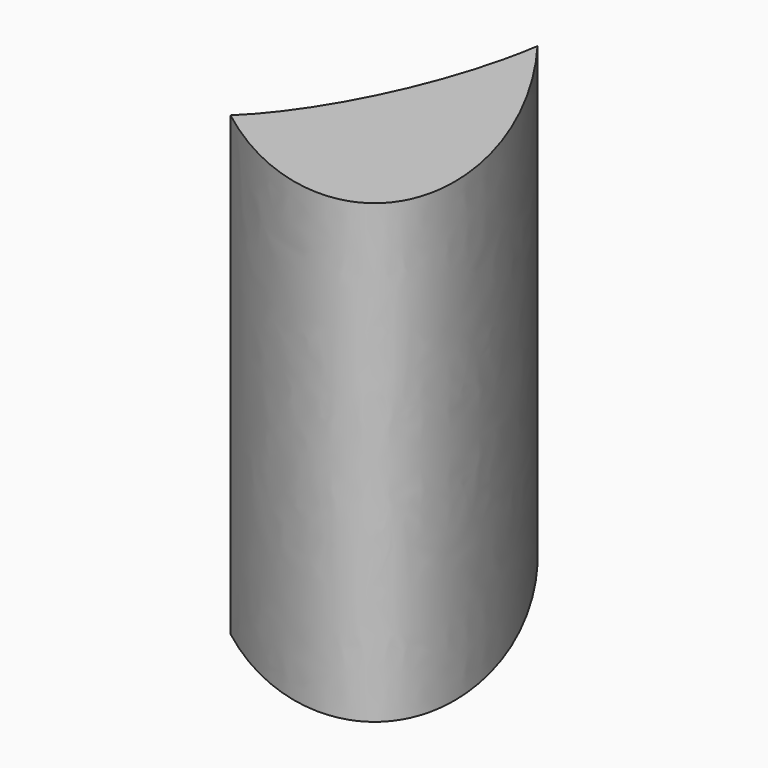
from build123d import *

# Parameters (mm, degrees)
F1_DEPTH = 127


with BuildPart() as f1:
    # F0 (on Top) → F1 (new body)
    with BuildSketch(Plane.XY):
        with BuildLine():
            add(Edge.make_bspline(
                [(22.6135193944, -57.7585702957), (47.7457317539, -33.6974171986), (54.3446338515, 9.3040225624)],
                knots=[0.7152454552, 0.7152454552, 0.7152454552, 2.048741235, 2.048741235, 2.048741235], degree=2, weights=[1, 0.7858370322, 1]))
            add(Edge.make_bspline(
                [(22.6135193944, -57.7585702957), (56.3772224768, -83.7389682514), (72.9023218155, -70.4779922962)],
                knots=[5.2078092816, 5.2078092816, 5.2078092816, 6.2831853072, 6.2831853072, 6.2831853072], degree=2, weights=[1, 0.8588950638, 1]))
            add(Edge.make_bspline(
                [(72.9023218155, -70.4779922962), (98.8890877871, -49.6242672057), (54.3446338515, 9.3040225624)],
                knots=[0, 0, 0, 1.5065215751, 1.5065215751, 1.5065215751], degree=2, weights=[1, 0.7294623037, 1]))
        make_face()
    extrude(amount=F1_DEPTH)


solid = f1.part
